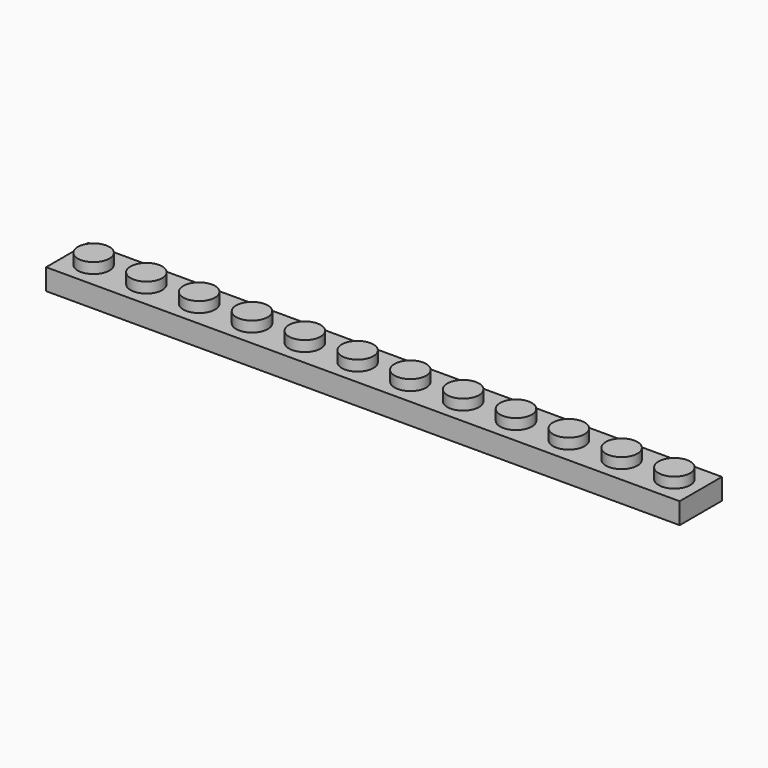
from build123d import *

# Parameters (mm, degrees)
F0_W     = 95.25
F0_H     = 7.9375
F0_R     = 2.38125
F1_DEPTH = 3.175
F2_DEPTH = 4.7625
F3_T     = -1.5875
F4_R     = 1.5875
F4_R_2   = 0.79375
F5_DEPTH = 1.5875


# Not quite as in the source:
# - a feature names something its author has since deleted; it is built from what else it names


with BuildPart() as f1:
    # F0 (on Top) → F1 (new body)
    with BuildSketch(Plane.XY):
        Rectangle(F0_W, F0_H)
        with Locations((-43.65625, 0)):
            Circle(F0_R, mode=Mode.SUBTRACT)
        with Locations((-35.71875, 0)):
            Circle(F0_R, mode=Mode.SUBTRACT)
        with Locations((-27.78125, 0)):
            Circle(F0_R, mode=Mode.SUBTRACT)
        with Locations((-19.84375, 0)):
            Circle(F0_R, mode=Mode.SUBTRACT)
        with Locations((-11.90625, 0)):
            Circle(F0_R, mode=Mode.SUBTRACT)
        with Locations((-3.96875, 0)):
            Circle(F0_R, mode=Mode.SUBTRACT)
        with Locations((3.96875, 0)):
            Circle(F0_R, mode=Mode.SUBTRACT)
        with Locations((11.90625, 0)):
            Circle(F0_R, mode=Mode.SUBTRACT)
        with Locations((19.84375, 0)):
            Circle(F0_R, mode=Mode.SUBTRACT)
        with Locations((27.78125, 0)):
            Circle(F0_R, mode=Mode.SUBTRACT)
        with Locations((35.71875, 0)):
            Circle(F0_R, mode=Mode.SUBTRACT)
        with Locations((43.65625, 0)):
            Circle(F0_R, mode=Mode.SUBTRACT)
    extrude(amount=F1_DEPTH)

    # F0 (on Top) → F2 (join)
    with BuildSketch(Plane.XY):
        with Locations((-43.65625, 0)):
            Circle(F0_R)
        with Locations((-27.78125, 0)):
            Circle(F0_R)
        with Locations((-35.71875, 0)):
            Circle(F0_R)
        with Locations((-19.84375, 0)):
            Circle(F0_R)
        with Locations((-11.90625, 0)):
            Circle(F0_R)
        with Locations((-3.96875, 0)):
            Circle(F0_R)
        with Locations((3.96875, 0)):
            Circle(F0_R)
        with Locations((11.90625, 0)):
            Circle(F0_R)
        with Locations((19.84375, 0)):
            Circle(F0_R)
        with Locations((27.78125, 0)):
            Circle(F0_R)
        with Locations((35.71875, 0)):
            Circle(F0_R)
        with Locations((43.65625, 0)):
            Circle(F0_R)
    extrude(amount=F2_DEPTH)

    # F3
    f3_openings = [f1.faces().sort_by_distance(p)[0] for p in [
        (0, 0, 0),
    ]]
    offset(amount=F3_T, openings=f3_openings, kind=Kind.INTERSECTION)

    # F4 (on face) → F5 (join)
    with BuildSketch(Plane(origin=(0, 0, 1.5875), x_dir=(1, 0, 0), z_dir=(0, 0, -1))):
        with Locations((-39.6875, 0)):
            Circle(F4_R)
        with Locations((-39.6875, 0)):
            Circle(F4_R_2, mode=Mode.SUBTRACT)
        with Locations((-31.75, 0)):
            Circle(F4_R)
        with Locations((-31.75, 0)):
            Circle(F4_R_2, mode=Mode.SUBTRACT)
        with Locations((-23.8125, 0)):
            Circle(F4_R)
        with Locations((-23.8125, 0)):
            Circle(F4_R_2, mode=Mode.SUBTRACT)
        with Locations((-15.875, 0)):
            Circle(F4_R)
        with Locations((-15.875, 0)):
            Circle(F4_R_2, mode=Mode.SUBTRACT)
        with Locations((-7.9375, 0)):
            Circle(F4_R)
        with Locations((-7.9375, 0)):
            Circle(F4_R_2, mode=Mode.SUBTRACT)
        Circle(F4_R)
        Circle(F4_R_2, mode=Mode.SUBTRACT)
        with Locations((7.9375, 0)):
            Circle(F4_R)
        with Locations((7.9375, 0)):
            Circle(F4_R_2, mode=Mode.SUBTRACT)
        with Locations((15.875, 0)):
            Circle(F4_R)
        with Locations((15.875, 0)):
            Circle(F4_R_2, mode=Mode.SUBTRACT)
        with Locations((23.8125, 0)):
            Circle(F4_R)
        with Locations((23.8125, 0)):
            Circle(F4_R_2, mode=Mode.SUBTRACT)
        with Locations((31.75, 0)):
            Circle(F4_R)
        with Locations((31.75, 0)):
            Circle(F4_R_2, mode=Mode.SUBTRACT)
        with Locations((39.6875, 0)):
            Circle(F4_R)
        with Locations((39.6875, 0)):
            Circle(F4_R_2, mode=Mode.SUBTRACT)
    extrude(amount=F5_DEPTH)


solid = f1.part
